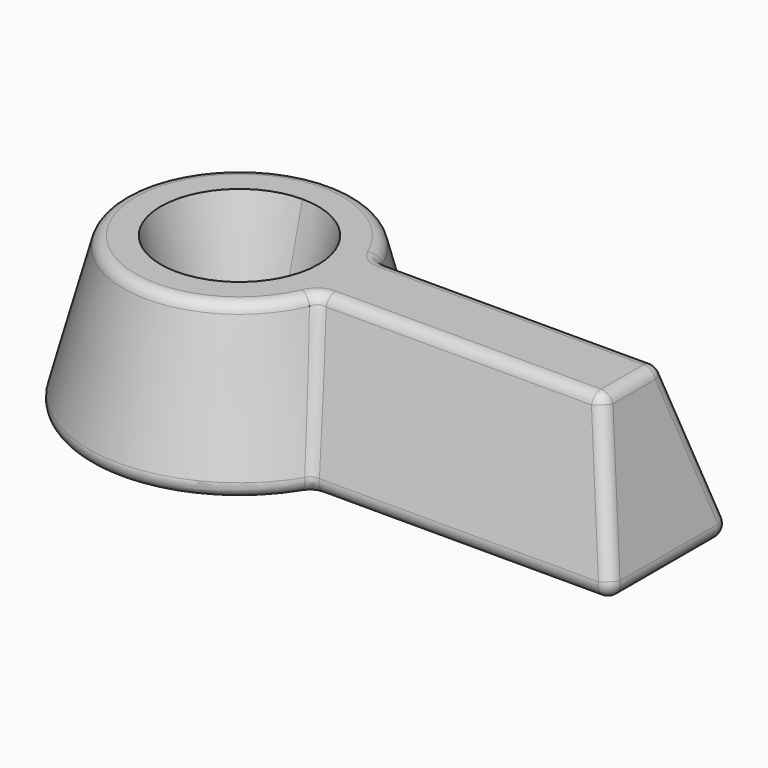
from build123d import *

# Parameters (mm, degrees)
F1_DEPTH               = 25
DRAFT_F1_DRAFTED_ANGLE = 15
F2_R                   = 2


# Not quite as in the source:
# - two fillets or chamfers of one size are made in one step
# - an extrude with a draft is written as a straight extrude whose walls are then drafted


with BuildPart() as f1:
    # F0 (on Top) → F1 (new body)
    with BuildSketch(Plane.XY):
        with BuildLine():
            ThreePointArc((21.6506350946, -12.5), (24.1481456572, -6.4704761276), (25, 0))
            ThreePointArc((25, 0), (24.1481456572, 6.4704761276), (21.6506350946, 12.5))
            Line((21.6506350946, 12.5), (0, 12.5))
            Line((0, 12.5), (0, 6))
            ThreePointArc((0, 6), (4.2426406871, 4.2426406871), (6, 0))
            ThreePointArc((6, 0), (4.2426406871, -4.2426406871), (0, -6))
            Line((0, -6), (0, -12.5))
            Line((0, -12.5), (21.6506350946, -12.5))
        make_face()
        with BuildLine():
            ThreePointArc((21.6506350946, 12.5), (24.1481456572, 6.4704761276), (25, 0))
            ThreePointArc((25, 0), (24.1481456572, -6.4704761276), (21.6506350946, -12.5))
            Line((21.6506350946, -12.5), (70, -12.5))
            Line((70, -12.5), (70, 12.5))
            Line((70, 12.5), (21.6506350946, 12.5))
        make_face()
        with BuildLine():
            Line((0, 12.5), (21.6506350946, 12.5))
            ThreePointArc((21.6506350946, 12.5), (-25, 0), (21.6506350946, -12.5))
            Line((21.6506350946, -12.5), (0, -12.5))
            Line((0, -12.5), (0, -6))
            ThreePointArc((0, -6), (-6, 0), (0, 6))
            Line((0, 6), (0, 12.5))
        make_face()
    extrude(amount=F1_DEPTH)

    # draft_F1_drafted
    draft_f1_drafted_walls = [f1.faces().sort_by_distance(p)[0] for p in [
        (0, 6, 16.6666666667),
        (45.8253175473, -12.5, 16.6666666667),
        (70, 0, 16.6666666667),
        (45.8253175473, 12.5, 16.6666666667),
        (-25, 0, 16.6666666667),
    ]]
    draft(draft_f1_drafted_walls, neutral_plane=Plane.XY, angle=DRAFT_F1_DRAFTED_ANGLE)

    # F2
    f2_edges = [f1.edges().sort_by_distance(p)[0] for p in [
        (19.504052, -8.966322, 13.187864),
        (66.650635, -9.150635, 12.5),
        (45.825318, -12.5, 0),
        (40.32937, -5.80127, 25),
        (66.650635, 9.150635, 12.5),
        (70, 0, 0),
        (63.30127, 0, 25),
        (19.504052, 8.966322, 13.187864),
        (45.825318, 12.5, 0),
        (40.32937, 5.80127, 25),
        (-25, 0, 0),
        (-18.30127, 0, 25),
    ]]
    fillet(f2_edges, radius=F2_R)


solid = f1.part
